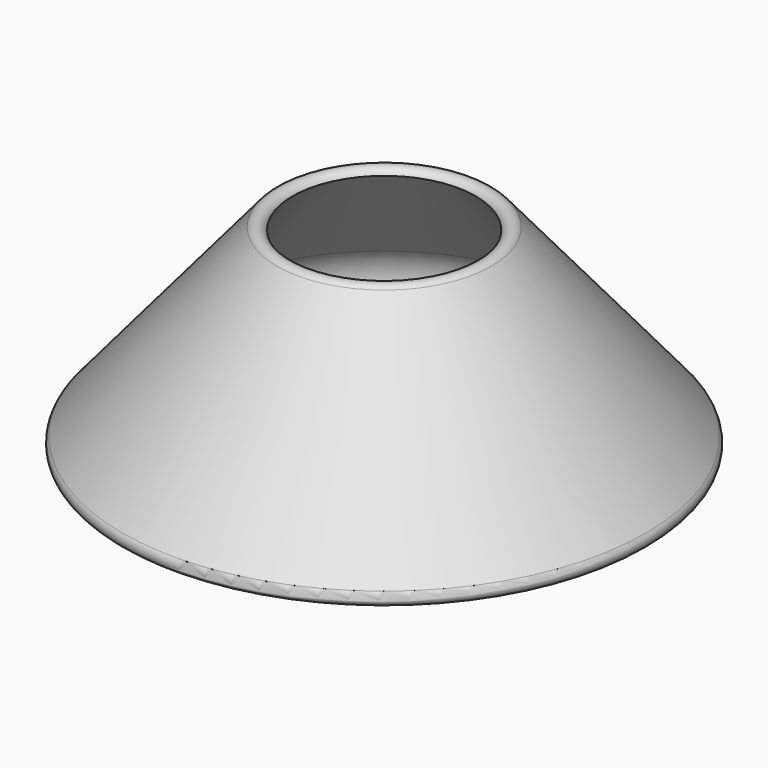
from build123d import *


# Not quite as in the source:
# - a fillet or chamfer that OpenCascade refuses, or shapes differently, is made with other operations: its cross-section is extruded or revolved along the edge and cut away or added


with BuildPart() as f1:
    # F0 (on Front) → F1 (revolve)
    with BuildSketch(Plane.XZ):
        Polygon((20, 1.5), (20, 0), (30, 0), (10, 23.8350718519), (10, 21.5014861116), (26.7832396192, 1.5), align=None)
    revolve(axis=Axis((0, 0, 12.1238185093), (0, 0, 1)))

    # F2: fillet of radius 5 on 1 edges, made by hand

    # F2_s1 → F2_t2 (revolve)
    with BuildSketch(Plane.XZ):
        with BuildLine():
            ThreePointArc((20.7691072795, 8.6673638222), (21.9103444044, 4.9199541008), (20, 1.5))
            Line((20, 1.5), (20.0612222987, 1.4209314845))
            ThreePointArc((20.0612222987, 1.4209314845), (23.3916198096, 1.4), (26.7832396192, 1.4))
            Line((26.7832396192, 1.4), (26.8598440635, 1.564278761))
            Line((26.8598440635, 1.564278761), (20.8457117239, 8.7316425831))
            Line((20.8457117239, 8.7316425831), (20.7691072795, 8.6673638222))
        make_face()
    revolve(axis=Axis((0, 0, 1.5), (0, 0, 1)))

    # F3: fillet of radius 1 on 2 edges, made by hand

    # F3_s1 → F3_t2 (revolve, cut)
    with BuildSketch(Plane.XZ):
        with BuildLine():
            ThreePointArc((27.8554930795, 0), (28.7618008665, 0.5773817383), (28.6215375226, 1.6427876097))
            Line((28.6215375226, 1.6427876097), (28.6368584115, 1.6556433619))
            Line((28.6368584115, 1.6556433619), (30.0153208889, 0.0128557522))
            Line((30.0153208889, 0.0128557522), (30, -0.02))
            Line((30, -0.02), (27.8554930795, -0.02))
            Line((27.8554930795, -0.02), (27.8554930795, 0))
        make_face()
    revolve(axis=Axis((0, 0, 0), (0, 0, 1)), mode=Mode.SUBTRACT)

    # F3_s3 → F3_t4 (revolve, cut)
    with BuildSketch(Plane.XZ):
        with BuildLine():
            ThreePointArc((11.7057370639, 21.802253578), (10.7660444431, 22.1442737213), (10, 21.5014861116))
            Line((10, 21.5014861116), (9.9812061476, 21.5083265145))
            ThreePointArc((9.9812061476, 21.5083265145), (9.98, 22.6682789817), (9.98, 23.8350718519))
            Line((9.98, 23.8350718519), (10.0153208889, 23.8479276041))
            Line((10.0153208889, 23.8479276041), (11.7210579528, 21.8151093301))
            Line((11.7210579528, 21.8151093301), (11.7057370639, 21.802253578))
        make_face()
    revolve(axis=Axis((0, 0, 23.8350718519), (0, 0, 1)), mode=Mode.SUBTRACT)


solid = f1.part
